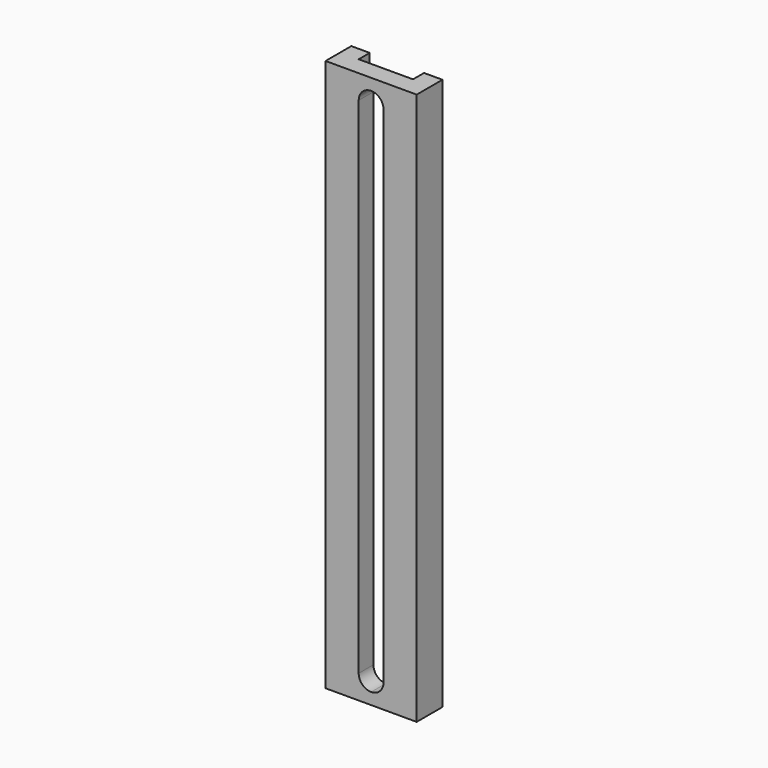
from build123d import *

# Parameters (mm, degrees)
F0_W     = 14.986
F0_H     = 152.4
F0_W_2   = 6.858
F0_H_2   = 146.05
F0_W_3   = 5.08
F1_DEPTH = 5.08
F2_R     = 3.42899
F3_DEPTH = 3.81


# Not quite as in the source:
# - a fillet or chamfer is up to 0.001 mm smaller than in the source, because OpenCascade refuses the exact size


with BuildPart() as f1:
    # F0 (on Front) → F1 (new body)
    with BuildSketch(Plane.XZ):
        Rectangle(F0_W, F0_H)
        Rectangle(F0_W_2, F0_H_2, mode=Mode.SUBTRACT)
        with Locations((-10.033, 0)):
            Rectangle(F0_W_3, F0_H)
        with Locations((10.033, 0)):
            Rectangle(F0_W_3, F0_H)
    extrude(amount=F1_DEPTH)

    # F2 (radius 3.429 in the source; OpenCascade refuses exactly that, so slightly less here)
    f2_edges = [f1.edges().sort_by_distance(p)[0] for p in [
        (3.429, -2.54, 73.025),
        (-3.429, -2.54, 73.025),
        (-3.429, -2.54, -73.025),
        (3.429, -2.54, -73.025),
    ]]
    fillet(f2_edges, radius=F2_R)

    # F0 (on Front) → F3 (join)
    with BuildSketch(Plane.XZ):
        with Locations((10.033, 0)):
            Rectangle(F0_W_3, F0_H)
        with Locations((-10.033, 0)):
            Rectangle(F0_W_3, F0_H)
    extrude(amount=-F3_DEPTH)


solid = f1.part
